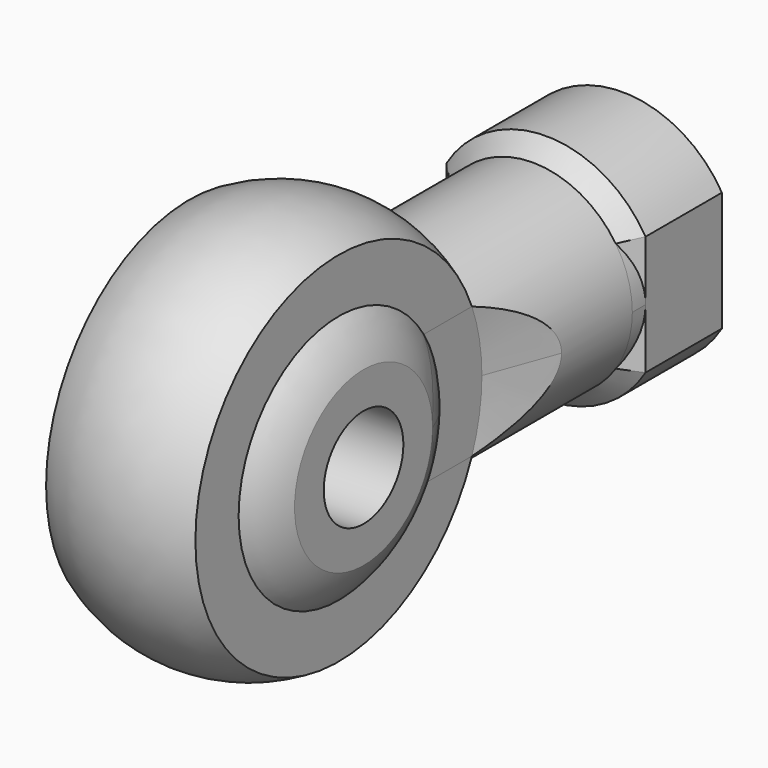
from build123d import *

# Parameters (mm, degrees)
F8_R          = 1.5
F10_DEPTH     = 3.375
F11_DEPTH     = 6
F12_T2_ANGLE  = 160.1226593158
F12_T6_DEPTH  = 3.0886171317
F12_S7_R      = 3
F12_T8_DEPTH  = 3
F12_T12_DEPTH = 3.0886171317
F12_S13_R     = 3
F12_T14_DEPTH = 3
F12_T16_ANGLE = 160.1226593158
F12_T20_DEPTH = 3.0886171317
F12_S21_R     = 3
F12_T22_DEPTH = 3
F12_T26_DEPTH = 3.0886171317
F12_S27_R     = 3
F12_T28_DEPTH = 3


# Not quite as in the source:
# - a fillet or chamfer that OpenCascade refuses, or shapes differently, is made with other operations: its cross-section is extruded or revolved along the edge and cut away or added


with BuildPart() as f6:
    # F5 (on Top) → F6 (revolve)
    with BuildSketch(Plane.XY):
        with BuildLine():
            Line((-3, 2.6), (-3, 1.5))
            Line((-3, 1.5), (3, 1.5))
            Line((3, 1.5), (3, 2.6))
            ThreePointArc((3, 2.6), (2.689266509, 3.2256435447), (2.25, 3.7688102609))
            ThreePointArc((2.25, 3.7688102609), (0, 4.6953090617), (-2.25, 3.7688102609))
            ThreePointArc((-2.25, 3.7688102609), (-2.689266509, 3.2256435447), (-3, 2.6))
        make_face()
        with BuildLine():
            Line((-2.25, 5.397114317), (-2.25, 3.7688102609))
            ThreePointArc((-2.25, 3.7688102609), (0, 4.6953090617), (2.25, 3.7688102609))
            Line((2.25, 3.7688102609), (2.25, 5.397114317))
            ThreePointArc((2.25, 5.397114317), (0, 6), (-2.25, 5.397114317))
        make_face()
    revolve(axis=Axis((0, 0, 0), (1, 0, 0)))

    # F8 (on offset) → F9 (join, up to the next surface of F6)
    with BuildSketch(Plane.XZ.offset(-13.5)):
        with BuildLine():
            ThreePointArc((-3, 0), (0, -3), (3, 0))
            ThreePointArc((3, 0), (0, 3), (-3, 0))
        make_face()
        Circle(F8_R, mode=Mode.SUBTRACT)
        Circle(F8_R)
    extrude(until=Until.NEXT)

    # F8 (on offset) → F10 (join)
    with BuildSketch(Plane.XZ.offset(-13.5)):
        with BuildLine():
            ThreePointArc((-3, 0), (0, 3), (3, 0))
            Line((3, 0), (3, 1.8027756377))
            ThreePointArc((3, 1.8027756377), (0, 3.5), (-3, 1.8027756377))
            Line((-3, 1.8027756377), (-3, 0))
        make_face()
        with BuildLine():
            Line((3, -1.8027756377), (3, 0))
            ThreePointArc((3, 0), (0, -3), (-3, 0))
            Line((-3, 0), (-3, -1.8027756377))
            ThreePointArc((-3, -1.8027756377), (0, -3.5), (3, -1.8027756377))
        make_face()
    extrude(amount=F10_DEPTH)

    # F8 (on offset) → F11 (cut)
    with BuildSketch(Plane.XZ.offset(-13.5)):
        Circle(F8_R)
    extrude(amount=F11_DEPTH, mode=Mode.SUBTRACT)

    # F12: chamfer of 0.5 on 6 edges, made by hand

    # F12_s1 → F12_t2 (revolve, cut)
    with BuildSketch(Plane(origin=(0, 0, 0), x_dir=(0, 1, 0), z_dir=(0.1725939358, 0, -0.9849930626))):
        Polygon((10.125, 3), (10.625, 3.5), (10.125, 3.5), align=None)
    revolve(axis=Axis((0, 10.125, 0), (0, -1, 0)), revolution_arc=F12_T2_ANGLE, mode=Mode.SUBTRACT)


with BuildPart() as f12_tool4:
    # F12_s5 → F12_t6 (new body)
    with BuildSketch(Plane.XY):
        Polygon((2.5, 10.125), (3, 10.625), (3, 10.125), align=None)
    extrude(amount=F12_T6_DEPTH)

    # F12_s7 → F12_t8 (cut, symmetric)
    with BuildSketch(Plane.XZ.offset(-10.4)):
        Circle(F12_S7_R)
    extrude(amount=F12_T8_DEPTH, both=True, mode=Mode.SUBTRACT)


with BuildPart() as f6_1:
    add(f6.part)

    # F12_t3: cut F12_tool4
    add(f12_tool4.part, mode=Mode.SUBTRACT)


with BuildPart() as f12_tool10:
    # F12_s11 → F12_t12 (new body)
    with BuildSketch(Plane.XY.offset(3.0886171317)):
        Polygon((-2.5, 10.125), (-3, 10.625), (-3, 10.125), align=None)
    extrude(amount=-F12_T12_DEPTH)

    # F12_s13 → F12_t14 (cut, symmetric)
    with BuildSketch(Plane.XZ.offset(-10.4)):
        Circle(F12_S13_R)
    extrude(amount=F12_T14_DEPTH, both=True, mode=Mode.SUBTRACT)


with BuildPart() as f6_2:
    add(f6_1.part)

    # F12_t9: cut F12_tool10
    add(f12_tool10.part, mode=Mode.SUBTRACT)

    # F12_s15 → F12_t16 (revolve, cut)
    with BuildSketch(Plane(origin=(0, 0, 0), x_dir=(0, 1, 0), z_dir=(-0.1725939358, 0, 0.9849930626))):
        Polygon((10.125, 3), (10.625, 3.5), (10.125, 3.5), align=None)
    revolve(axis=Axis((0, 10.125, 0), (0, -1, 0)), revolution_arc=F12_T16_ANGLE, mode=Mode.SUBTRACT)


with BuildPart() as f12_tool18:
    # F12_s19 → F12_t20 (new body)
    with BuildSketch(Plane.XY.offset(-3.0886171317)):
        Polygon((2.5, 10.125), (3, 10.625), (3, 10.125), align=None)
    extrude(amount=F12_T20_DEPTH)

    # F12_s21 → F12_t22 (cut, symmetric)
    with BuildSketch(Plane.XZ.offset(-10.4)):
        Circle(F12_S21_R)
    extrude(amount=F12_T22_DEPTH, both=True, mode=Mode.SUBTRACT)


with BuildPart() as f6_3:
    add(f6_2.part)

    # F12_t17: cut F12_tool18
    add(f12_tool18.part, mode=Mode.SUBTRACT)


with BuildPart() as f12_tool24:
    # F12_s25 → F12_t26 (new body)
    with BuildSketch(Plane.XY):
        Polygon((-2.5, 10.125), (-3, 10.625), (-3, 10.125), align=None)
    extrude(amount=-F12_T26_DEPTH)

    # F12_s27 → F12_t28 (cut, symmetric)
    with BuildSketch(Plane.XZ.offset(-10.4)):
        Circle(F12_S27_R)
    extrude(amount=F12_T28_DEPTH, both=True, mode=Mode.SUBTRACT)


with BuildPart() as f6_4:
    add(f6_3.part)

    # F12_t23: cut F12_tool24
    add(f12_tool24.part, mode=Mode.SUBTRACT)

    # F5 (on Top) → F13 (revolve, cut)
    with BuildSketch(Plane.XY):
        with BuildLine():
            Line((3, 2.6), (3, 1.5))
            Line((3, 1.5), (5, 1.5))
            Line((5, 1.5), (5, 8.25))
            Line((5, 8.25), (3.2883654704, 8.25))
            Line((3.2883654704, 8.25), (2.25, 5.397114317))
            Line((2.25, 5.397114317), (2.25, 3.7688102609))
            ThreePointArc((2.25, 3.7688102609), (2.689266509, 3.2256435447), (3, 2.6))
        make_face()
        with BuildLine():
            Line((-5, 1.5), (-3, 1.5))
            Line((-3, 1.5), (-3, 2.6))
            ThreePointArc((-3, 2.6), (-2.689266509, 3.2256435447), (-2.25, 3.7688102609))
            Line((-2.25, 3.7688102609), (-2.25, 5.397114317))
            Line((-2.25, 5.397114317), (-3.2883654704, 8.25))
            Line((-3.2883654704, 8.25), (-5, 8.25))
            Line((-5, 8.25), (-5, 1.5))
        make_face()
    revolve(axis=Axis((0, 0, 0), (1, 0, 0)), mode=Mode.SUBTRACT)


solid = f6_4.part
